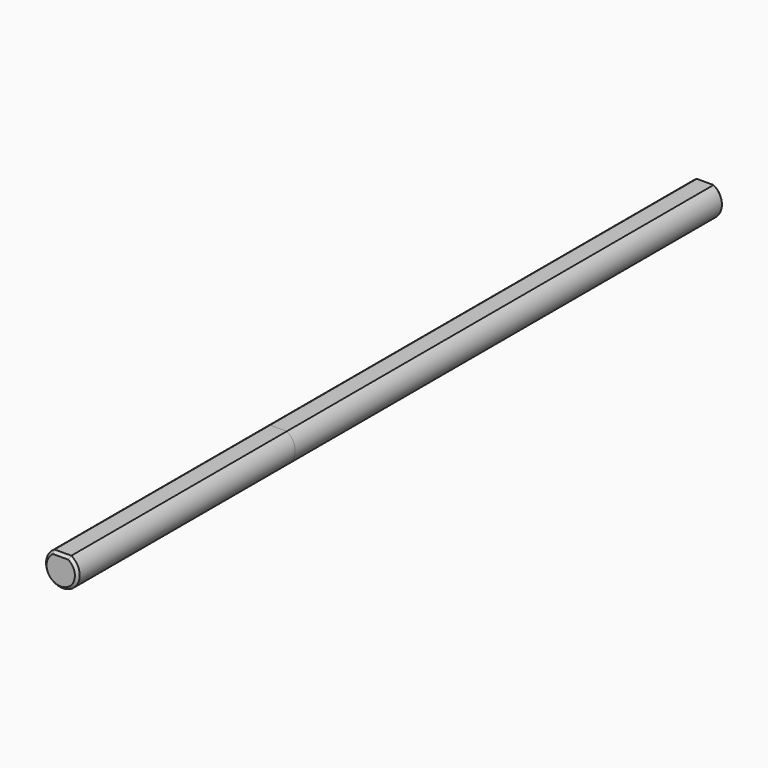
from build123d import *

# Parameters (mm, degrees)
F1_DEPTH     = 152.4
F2_DEPTH     = 76.2
F3_DEPTH     = 101.6
F4_C1_SIZE   = 0.508
F4_C2_SIZE   = 0.508
F4_C3_SIZE   = 0.508
F4_C4_SIZE   = 0.508
F4_2_C1_SIZE = 0.508
F4_2_C2_SIZE = 0.508
F4_2_C3_SIZE = 0.508
F4_2_C4_SIZE = 0.508
F4_3_C1_SIZE = 0.508
F4_3_C2_SIZE = 0.508
F4_3_C3_SIZE = 0.508
F4_3_C4_SIZE = 0.508


with BuildPart() as f1:
    # F0 (on Front) → F1 (new body)
    with BuildSketch(Plane.XZ):
        with BuildLine():
            Line((1.5875, 2.749630657), (-1.5875, 2.749630657))
            ThreePointArc((-1.5875, 2.749630657), (0, -3.175), (1.5875, 2.749630657))
        make_face()
    extrude(amount=F1_DEPTH)

    # F4: chamfer of 0.508 on 4 edges, made by hand

    # F4_c1
    f4_c1_edges = [f1.edges().sort_by_distance(p)[0] for p in [
        (0, 0, 2.749630657),
    ]]
    chamfer(f4_c1_edges, length=F4_C1_SIZE)

    # F4_c2
    f4_c2_edges = [f1.edges().sort_by_distance(p)[0] for p in [
        (0, -152.4, 2.749630657),
    ]]
    chamfer(f4_c2_edges, length=F4_C2_SIZE)

    # F4_c3
    f4_c3_edges = [f1.edges().sort_by_distance(p)[0] for p in [
        (0, 0, -3.175),
    ]]
    chamfer(f4_c3_edges, length=F4_C3_SIZE)

    # F4_c4
    f4_c4_edges = [f1.edges().sort_by_distance(p)[0] for p in [
        (0, -152.4, -3.175),
    ]]
    chamfer(f4_c4_edges, length=F4_C4_SIZE)


with BuildPart() as f2:
    # F0 (on Front) → F2 (new body)
    with BuildSketch(Plane.XZ):
        with BuildLine():
            Line((1.5875, 2.749630657), (-1.5875, 2.749630657))
            ThreePointArc((-1.5875, 2.749630657), (0, -3.175), (1.5875, 2.749630657))
        make_face()
    extrude(amount=F2_DEPTH)

    # F4#2: chamfer of 0.508 on 4 edges, made by hand

    # F4_2_c1
    f4_2_c1_edges = [f2.edges().sort_by_distance(p)[0] for p in [
        (0, 0, 2.749630657),
    ]]
    chamfer(f4_2_c1_edges, length=F4_2_C1_SIZE)

    # F4_2_c2
    f4_2_c2_edges = [f2.edges().sort_by_distance(p)[0] for p in [
        (0, -76.2, 2.749630657),
    ]]
    chamfer(f4_2_c2_edges, length=F4_2_C2_SIZE)

    # F4_2_c3
    f4_2_c3_edges = [f2.edges().sort_by_distance(p)[0] for p in [
        (0, 0, -3.175),
    ]]
    chamfer(f4_2_c3_edges, length=F4_2_C3_SIZE)

    # F4_2_c4
    f4_2_c4_edges = [f2.edges().sort_by_distance(p)[0] for p in [
        (0, -76.2, -3.175),
    ]]
    chamfer(f4_2_c4_edges, length=F4_2_C4_SIZE)


with BuildPart() as f3:
    # F0 (on Front) → F3 (new body)
    with BuildSketch(Plane.XZ):
        with BuildLine():
            Line((1.5875, 2.749630657), (-1.5875, 2.749630657))
            ThreePointArc((-1.5875, 2.749630657), (0, -3.175), (1.5875, 2.749630657))
        make_face()
    extrude(amount=F3_DEPTH)

    # F4#3: chamfer of 0.508 on 4 edges, made by hand

    # F4_3_c1
    f4_3_c1_edges = [f3.edges().sort_by_distance(p)[0] for p in [
        (0, 0, 2.749630657),
    ]]
    chamfer(f4_3_c1_edges, length=F4_3_C1_SIZE)

    # F4_3_c2
    f4_3_c2_edges = [f3.edges().sort_by_distance(p)[0] for p in [
        (0, -101.6, 2.749630657),
    ]]
    chamfer(f4_3_c2_edges, length=F4_3_C2_SIZE)

    # F4_3_c3
    f4_3_c3_edges = [f3.edges().sort_by_distance(p)[0] for p in [
        (0, 0, -3.175),
    ]]
    chamfer(f4_3_c3_edges, length=F4_3_C3_SIZE)

    # F4_3_c4
    f4_3_c4_edges = [f3.edges().sort_by_distance(p)[0] for p in [
        (0, -101.6, -3.175),
    ]]
    chamfer(f4_3_c4_edges, length=F4_3_C4_SIZE)


solid = Compound([f1.part, f2.part, f3.part])
